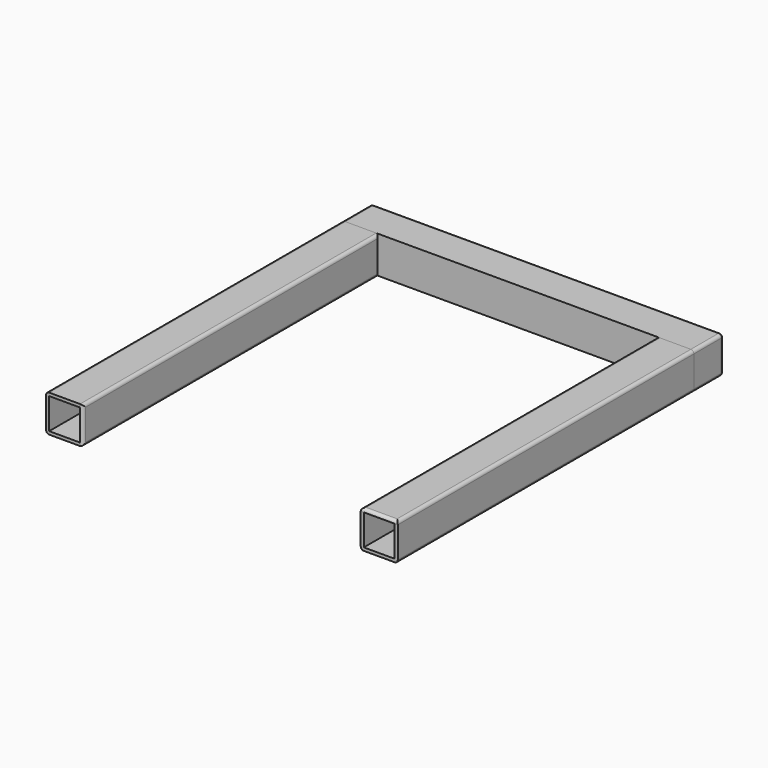
from build123d import *

# Parameters (mm, degrees)
F0_W     = 60
F0_H     = 60
F0_W_2   = 50
F0_H_2   = 50
F1_DEPTH = 600
F2_W     = 60
F2_H     = 60
F3_DEPTH = 285
F4_R     = 4.99999
F4_2_R   = 4.99999
F4_3_R   = 4.99999


# Not quite as in the source:
# - a fillet or chamfer is up to 0.001 mm smaller than in the source, because OpenCascade refuses the exact size


with BuildPart() as f1:
    # F0 (on Front) → F1 (new body)
    with BuildSketch(Plane.XZ):
        with Locations((255, 30)):
            Rectangle(F0_W, F0_H)
        with Locations((255, 30)):
            Rectangle(F0_W_2, F0_H_2, mode=Mode.SUBTRACT)
    extrude(amount=F1_DEPTH)

    # F4#3 (radius 5 in the source; OpenCascade refuses exactly that, so slightly less here)
    f4_3_edges = [f1.edges().sort_by_distance(p)[0] for p in [
        (225, -300, 60),
        (255, -600, 60),
        (285, -300, 60),
        (285, -300, 0),
        (225, -300, 0),
    ]]
    fillet(f4_3_edges, radius=F4_3_R)


with BuildPart() as f1b:
    # F0 (on Front) → F1, piece 2 (new body)
    with BuildSketch(Plane.XZ):
        with Locations((-255, 30)):
            Rectangle(F0_W, F0_H)
        with Locations((-255, 30)):
            Rectangle(F0_W_2, F0_H_2, mode=Mode.SUBTRACT)
    extrude(amount=F1_DEPTH)

    # F4#2 (radius 5 in the source; OpenCascade refuses exactly that, so slightly less here)
    f4_2_edges = [f1b.edges().sort_by_distance(p)[0] for p in [
        (-225, -300, 0),
        (-225, -300, 60),
        (-225, 0, 30),
        (-225, -600, 30),
        (-285, -300, 60),
        (-285, -300, 0),
    ]]
    fillet(f4_2_edges, radius=F4_2_R)


with BuildPart() as f3:
    # F2 (on Right) → F3 (new body, symmetric)
    with BuildSketch(Plane.YZ):
        with Locations((30, 30)):
            Rectangle(F2_W, F2_H)
    extrude(amount=F3_DEPTH, both=True)

    # F4 (radius 5 in the source; OpenCascade refuses exactly that, so slightly less here)
    f4_edges = [f3.edges().sort_by_distance(p)[0] for p in [
        (-285, 60, 30),
        (0, 60, 60),
        (285, 60, 30),
        (0, 60, 0),
        (-285, 30, 60),
        (-285, 30, 0),
        (285, 30, 60),
        (285, 30, 0),
    ]]
    fillet(f4_edges, radius=F4_R)


solid = Compound([f1.part, f1b.part, f3.part])
